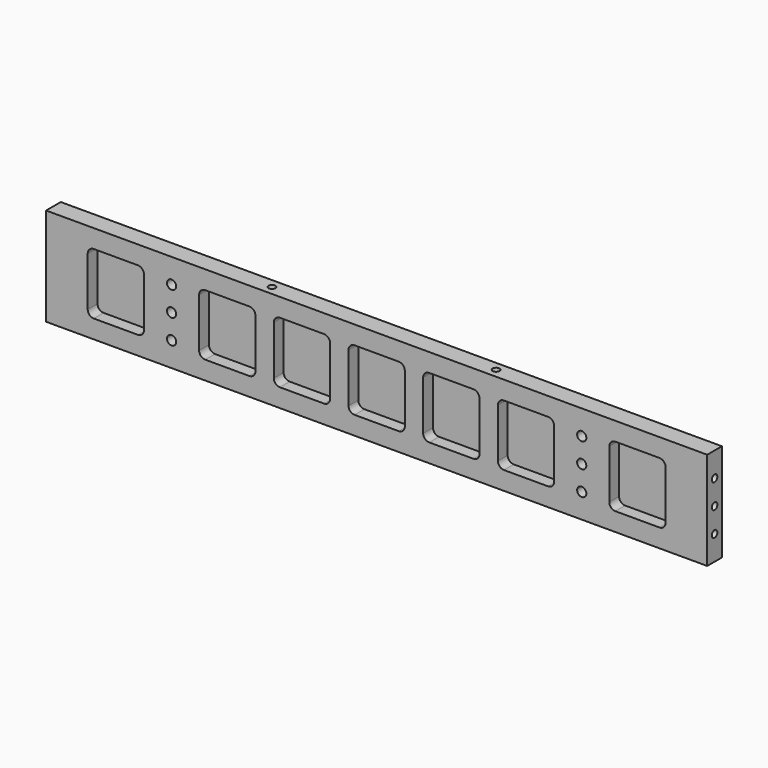
from build123d import *

# Parameters (mm, degrees)
F0_W             = 342.9
F0_H             = 50.8
F1_DEPTH         = 9.525
F2_D             = 4.7625
F2_CSINK_D       = 10.16
F2_CSINK_ANGLE   = 90
F4_D             = 3.571875
F4_DEPTH         = 12.7
F4_TIP           = 1.0730995118
F6_D             = 3.571875
F6_DEPTH         = 12.7
F6_TIP           = 1.0730995118
F7_W             = 29.21
F7_H             = 31.75
F8_DEPTH         = 6.35
F9_R             = 3.175
F12_D            = 3.571875
F12_DEPTH        = 6.35
F12_TIP          = 1.0730995118
F12_ON_F10_D     = 3.571875
F12_ON_F10_DEPTH = 6.35
F12_ON_F10_TIP   = 1.0730995118


# Not quite as in the source:
# - a feature names something its author has since deleted; it is built from what else it names


with BuildPart() as f1:
    # F0 (on Front) → F1 (new body)
    with BuildSketch(Plane.XZ):
        with Locations((171.45, 25.4)):
            Rectangle(F0_W, F0_H)
    extrude(amount=F1_DEPTH)

    # F2 (through all)
    with Locations(Plane(origin=(0, 0, 0), x_dir=(1, 0, 0), z_dir=(0, 1, 0))):
        with Locations((65.0875, -38.1), (65.0875, -25.4), (65.0875, -12.7), (277.8125, -38.1), (277.8125, -25.4), (277.8125, -12.7)):
            CounterSinkHole(F2_D / 2, F2_CSINK_D / 2, counter_sink_angle=F2_CSINK_ANGLE)

    # F4
    with Locations(Plane(origin=(0, 0, 0), x_dir=(0, -1, 0), z_dir=(-1, 0, 0))):
        with Locations((4.7625, 25.4), (4.7625, 12.7), (4.7625, 38.1)):
            Hole(F4_D / 2, depth=F4_DEPTH)
            with Locations((0, 0, -(F4_DEPTH + F4_TIP / 2))):  # 118° drill point
                Cone(0, F4_D / 2, F4_TIP, mode=Mode.SUBTRACT)

    # F6
    with Locations(Plane.YZ.offset(342.9)):
        with Locations((-4.7625, 12.7), (-4.7625, 25.4), (-4.7625, 38.1)):
            Hole(F6_D / 2, depth=F6_DEPTH)
            with Locations((0, 0, -(F6_DEPTH + F6_TIP / 2))):  # 118° drill point
                Cone(0, F6_D / 2, F6_TIP, mode=Mode.SUBTRACT)

    # F7 (on face) → F8 (cut)
    with BuildSketch(Plane.XZ.offset(9.525)):
        with Locations((93.98, 25.4)):
            Rectangle(F7_W, F7_H)
        with Locations((132.715, 25.4)):
            Rectangle(F7_W, F7_H)
        with Locations((171.45, 25.4)):
            Rectangle(F7_W, F7_H)
        with Locations((210.185, 25.4)):
            Rectangle(F7_W, F7_H)
        with Locations((248.92, 25.4)):
            Rectangle(F7_W, F7_H)
        with Locations((36.195, 25.4)):
            Rectangle(F7_W, F7_H)
        with Locations((306.705, 25.4)):
            Rectangle(F7_W, F7_H)
    extrude(amount=-F8_DEPTH, mode=Mode.SUBTRACT)

    # F9
    f9_edges = [f1.edges().sort_by_distance(p)[0] for p in [
        (156.845, -6.35, 41.275),
        (195.58, -6.35, 41.275),
        (234.315, -6.35, 41.275),
        (79.375, -6.35, 41.275),
        (118.11, -6.35, 41.275),
        (79.375, -6.35, 9.525),
        (118.11, -6.35, 9.525),
        (156.845, -6.35, 9.525),
        (195.58, -6.35, 9.525),
        (234.315, -6.35, 9.525),
        (108.585, -6.35, 41.275),
        (147.32, -6.35, 41.275),
        (186.055, -6.35, 41.275),
        (224.79, -6.35, 41.275),
        (263.525, -6.35, 41.275),
        (263.525, -6.35, 9.525),
        (224.79, -6.35, 9.525),
        (186.055, -6.35, 9.525),
        (147.32, -6.35, 9.525),
        (108.585, -6.35, 9.525),
        (321.31, -6.35, 41.275),
        (292.1, -6.35, 41.275),
        (292.1, -6.35, 9.525),
        (321.31, -6.35, 9.525),
        (50.8, -6.35, 9.525),
        (50.8, -6.35, 41.275),
        (21.59, -6.35, 41.275),
        (21.59, -6.35, 9.525),
    ]]
    fillet(f9_edges, radius=F9_R)

    # F12
    with Locations(Plane.XY.offset(50.8)):
        with Locations((229.5525, -4.7625), (113.3475, -4.7625)):
            Hole(F12_D / 2, depth=F12_DEPTH)
            with Locations((0, 0, -(F12_DEPTH + F12_TIP / 2))):  # 118° drill point
                Cone(0, F12_D / 2, F12_TIP, mode=Mode.SUBTRACT)

    # F12 on F10
    with Locations(Plane(origin=(0, 0, 0), x_dir=(1, 0, 0), z_dir=(0, 0, -1))):
        with Locations((113.3475, 4.7625), (229.5525, 4.7625)):
            Hole(F12_ON_F10_D / 2, depth=F12_ON_F10_DEPTH)
            with Locations((0, 0, -(F12_ON_F10_DEPTH + F12_ON_F10_TIP / 2))):  # 118° drill point
                Cone(0, F12_ON_F10_D / 2, F12_ON_F10_TIP, mode=Mode.SUBTRACT)


solid = f1.part
